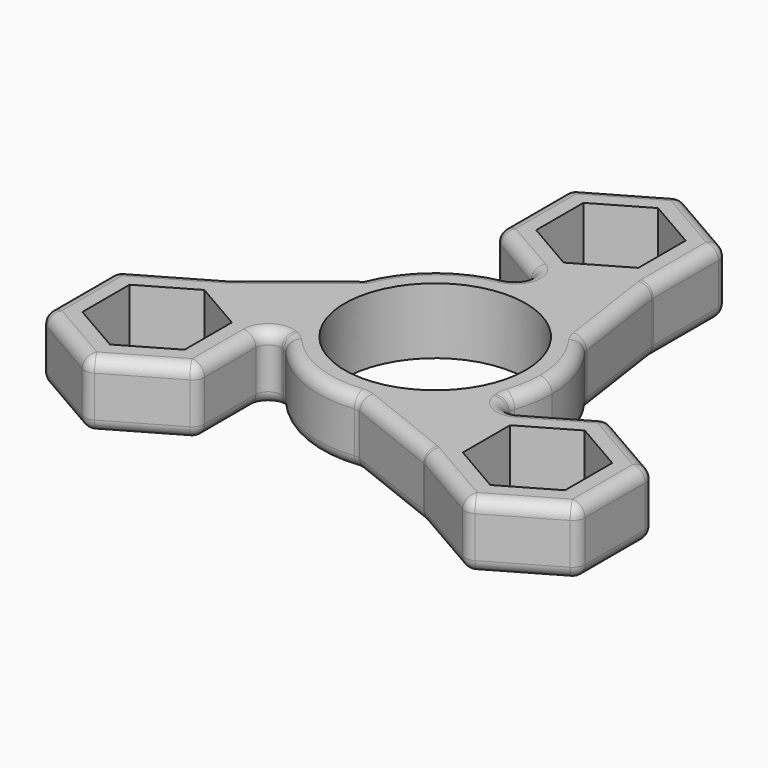
from build123d import *

# Parameters (mm, degrees)
F0_R     = 10.975
F1_DEPTH = 4
F2_F1_R  = 1.5
F2_F2_R  = 1.5


with BuildPart() as f1:
    # F0 (on Top) → F1 (new body, symmetric)
    with BuildSketch(Plane.XY):
        with BuildLine():
            Line((11.2497384604, 8.624036733), (9.4, 21.2187224089))
            Line((9.4, 21.2187224089), (0, 15.7916298785))
            Line((0, 15.7916298785), (-2.2752234976, 13.991210921))
            ThreePointArc((-2.2752234976, 13.991210921), (5.2284911204, 13.1754888184), (11.2497384604, 8.624036733))
        make_face()
        Polygon((0, 15.7916298785), (9.4, 21.2187224089), (9.4, 32.0729074696), (0, 37.5), (-9.4, 32.0729074696), (-9.4, 21.2187224089), align=None)
        Polygon((6.2, 30.2253866082), (6.2, 23.0662432703), (0, 19.4866716013), (-6.2, 23.0662432703), (-6.2, 30.2253866082), (0, 33.8049582772), align=None, mode=Mode.SUBTRACT)
        with BuildLine():
            Line((13.2543558361, -5.0252041123), (11.2497384604, 8.624036733))
            ThreePointArc((11.2497384604, 8.624036733), (5.2284911204, 13.1754888184), (-2.2752234976, 13.991210921))
            Line((-2.2752234976, 13.991210921), (-13.0935041242, 5.4305409261))
            ThreePointArc((-13.0935041242, 5.4305409261), (-14.0245535842, -2.0597382755), (-10.9791323385, -8.9660068087))
            Line((-10.9791323385, -8.9660068087), (1.8437656638, -14.0545776592))
            ThreePointArc((1.8437656638, -14.0545776592), (8.7960624639, -11.1157505429), (13.2543558361, -5.0252041123))
        make_face()
        Circle(F0_R, mode=Mode.SUBTRACT)
        with BuildLine():
            ThreePointArc((14.175, 0), (13.4237786721, 4.5533274824), (11.2497384604, 8.624036733))
            Line((11.2497384604, 8.624036733), (13.2543558361, -5.0252041123))
            ThreePointArc((13.2543558361, -5.0252041123), (13.9429394135, -2.5544207781), (14.175, 0))
        make_face()
        with BuildLine():
            Line((-13.0935041242, 5.4305409261), (-2.2752234976, 13.991210921))
            ThreePointArc((-2.2752234976, 13.991210921), (-8.7960624639, 11.1157505429), (-13.0935041242, 5.4305409261))
        make_face()
        with BuildLine():
            Line((13.6759526419, -7.8958149392), (13.2543558361, -5.0252041123))
            ThreePointArc((13.2543558361, -5.0252041123), (8.7960624639, -11.1157505429), (1.8437656638, -14.0545776592))
            Line((1.8437656638, -14.0545776592), (13.6759526419, -18.75))
            Line((13.6759526419, -18.75), (13.6759526419, -7.8958149392))
        make_face()
        with BuildLine():
            ThreePointArc((-10.9791323385, -8.9660068087), (-14.0245535842, -2.0597382755), (-13.0935041242, 5.4305409261))
            Line((-13.0935041242, 5.4305409261), (-23.0759526419, -2.4687224089))
            Line((-23.0759526419, -2.4687224089), (-13.6759526419, -7.8958149392))
            Line((-13.6759526419, -7.8958149392), (-10.9791323385, -8.9660068087))
        make_face()
        with BuildLine():
            ThreePointArc((-10.9791323385, -8.9660068087), (-5.2284911204, -13.1754888184), (1.8437656638, -14.0545776592))
            Line((1.8437656638, -14.0545776592), (-10.9791323385, -8.9660068087))
        make_face()
        Polygon((23.0759526419, -2.4687224089), (13.6759526419, -7.8958149392), (13.6759526419, -18.75), (23.0759526419, -24.1770925304), (32.4759526419, -18.75), (32.4759526419, -7.8958149392), align=None)
        Polygon((29.2759526419, -9.7433358006), (29.2759526419, -16.9024791386), (23.0759526419, -20.4820508076), (16.8759526419, -16.9024791386), (16.8759526419, -9.7433358006), (23.0759526419, -6.1637641317), align=None, mode=Mode.SUBTRACT)
        Polygon((-13.6759526419, -7.8958149392), (-23.0759526419, -2.4687224089), (-32.4759526419, -7.8958149392), (-32.4759526419, -18.75), (-23.0759526419, -24.1770925304), (-13.6759526419, -18.75), align=None)
        Polygon((-16.8759526419, -9.7433358006), (-16.8759526419, -16.9024791386), (-23.0759526419, -20.4820508076), (-29.2759526419, -16.9024791386), (-29.2759526419, -9.7433358006), (-23.0759526419, -6.1637641317), align=None, mode=Mode.SUBTRACT)
    extrude(amount=F1_DEPTH, both=True)

    # F2: fillet of radius 1.5 on 55 edges, made by hand

    # F2_f1
    f2_f1_edges = [f1.edges().sort_by_distance(p)[0] for p in [
        (-13.6759526419, -7.8958149392, 0),
        (-10.9791323385, -8.9660068087, 0),
        (1.8437656638, -14.0545776592, 0),
        (13.6759526419, -18.75, 0),
        (13.6759526419, -7.8958149392, 0),
        (13.2543558361, -5.0252041123, 0),
        (9.4, 21.2187224089, 0),
        (11.2497384604, 8.624036733, 0),
        (0, 15.7916298785, 0),
        (-2.2752234976, 13.991210921, 0),
        (-23.0759526419, -2.4687224089, 0),
    ]]
    fillet(f2_f1_edges, radius=F2_F1_R)

    # F2_f2
    f2_f2_edges = [f1.edges().sort_by_distance(p)[0] for p in [
        (-23.0759526419, -24.1770925304, 0),
        (-18.3759526419, -21.4635462652, -4),
        (-13.6759526419, -18.75, 0),
        (-18.3759526419, -21.4635462652, 4),
        (7.8851542245, -16.4520102614, -4),
        (7.8851542245, -16.4520102614, 4),
        (23.0759526419, -24.1770925304, 0),
        (27.7759526419, -21.4635462652, -4),
        (32.4759526419, -18.75, 0),
        (27.7759526419, -21.4635462652, 4),
        (32.4759526419, -13.3229074696, -4),
        (32.4759526419, -7.8958149392, 0),
        (32.4759526419, -13.3229074696, 4),
        (27.7759526419, -5.182268674, -4),
        (23.0759526419, -2.4687224089, 0),
        (27.7759526419, -5.182268674, 4),
        (13.3322061894, -5.5552794447, -4),
        (13.3322061894, -5.5552794447, 4),
        (10.3052817175, 15.0547490019, -4),
        (10.3052817175, 15.0547490019, 4),
        (0, 37.5, 0),
        (-4.7, 34.7864537348, -4),
        (-9.4, 32.0729074696, 0),
        (-4.7, 34.7864537348, 4),
        (9.4, 32.0729074696, 0),
        (4.7, 34.7864537348, -4),
        (4.7, 34.7864537348, 4),
        (-1.8550899705, 14.3236689708, -4),
        (-1.8550899705, 14.3236689708, 4),
        (-9.4, 26.6458149392, -4),
        (-9.4, 21.2187224089, 0),
        (-9.4, 26.6458149392, 4),
        (-27.8233945012, -5.2096592443, -4),
        (-32.4759526419, -7.8958149392, 0),
        (-27.8233945012, -5.2096592443, 4),
        (-32.4759526419, -13.3229074696, -4),
        (-32.4759526419, -18.75, 0),
        (-32.4759526419, -13.3229074696, 4),
        (-27.7759526419, -21.4635462652, -4),
        (-27.7759526419, -21.4635462652, 4),
        (-23.0781974181, -2.4654165357, 4),
        (-23.0781974181, -2.4654165357, -4),
        (-1.1670737223, 15.7063850391, 4),
        (-2.2860682382, 14.0380882713, 4),
        (-1.1670737223, 15.7063850391, -4),
        (-2.2860682382, 14.0380882713, -4),
        (11.2897755602, 8.6507224036, 4),
        (9.4039853583, 21.2190135055, 4),
        (11.2897755602, 8.6507224036, -4),
        (9.4039853583, 21.2190135055, -4),
        (14.1856653066, -6.842477028, 4),
        (13.3003751826, -5.0392509666, 4),
        (14.1856653066, -6.842477028, -4),
        (13.3003751826, -5.0392509666, -4),
        (1.8468575825, -14.1025936399, 4),
        (13.6742120599, -18.7535969698, 4),
        (1.8468575825, -14.1025936399, -4),
        (13.6742120599, -18.7535969698, -4),
    ]]
    fillet(f2_f2_edges, radius=F2_F2_R)


solid = f1.part
